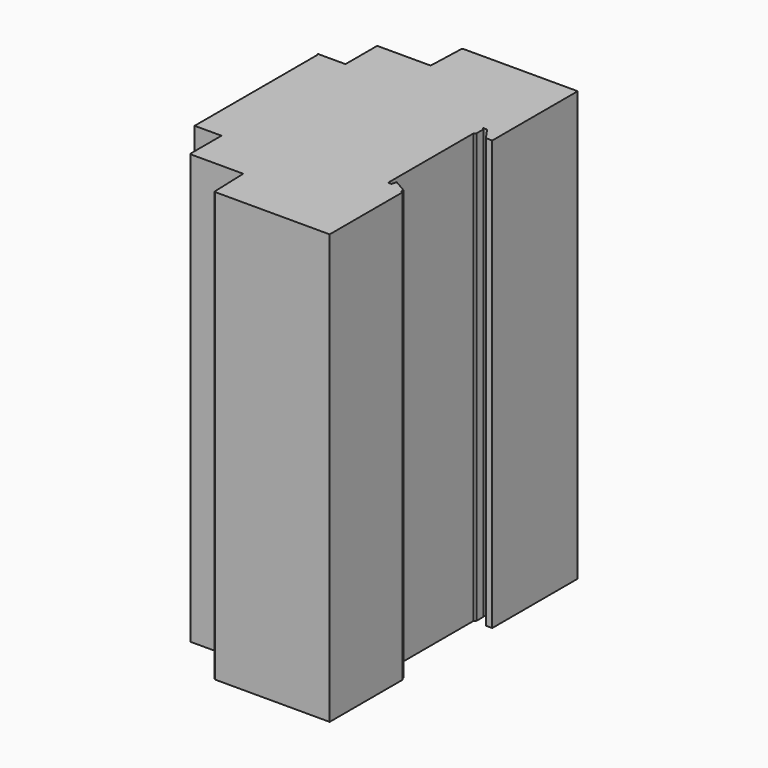
from build123d import *

# Parameters (mm, degrees)
F1_DEPTH = 124.6
F2_R     = 0.25
F3_R     = 2.1
F4_R     = 2.1
F6_DEPTH = 16
F5_W     = 44.5
F5_H     = 124.6
F5_W_2   = 30.3
F5_H_2   = 57.1
F5_R     = 3.57
F5_R_2   = 1
F5_W_3   = 24
F5_H_3   = 48
F5_R_3   = 2.35
F7_DEPTH = 0.2
F8_DEPTH = 0.5
F9_DEPTH = 0.1
F10_R    = 0.1


# Not quite as in the source:
# - ends of sketch curves that miss each other by under 0.0002 mm in the source are joined


with BuildPart() as f1:
    # F0 (on Top) → F1 (new body)
    with BuildSketch(Plane.XY):
        with BuildLine():
            ThreePointArc((-15.8128712425, -37.7039390085), (-15.7214514538, -37.9092709955), (-15.513054, -37.993469))
            Line((-15.513054, -37.993469), (4.69724, -37.993469))
            Line((4.69724, -37.993469), (5.19724, -37.993469))
            Line((5.19724, -37.993469), (17.69724, -37.993469))
            Line((17.69724, -37.993469), (17.69724, -11.597317))
            Line((17.69724, -11.597317), (17.19724, -11.463342))
            Line((17.19724, -11.463342), (17.19724, -10.586289))
            Line((17.19724, -10.586289), (13.572369, -8.493469))
            Line((13.572369, -8.493469), (13.19724, -9.893469))
            Line((13.19724, -9.893469), (12.19724, -9.893469))
            Line((12.19724, -9.893469), (12.19724, 21.006531))
            Line((12.19724, 21.006531), (12.69724, 21.506531))
            Line((12.69724, 21.506531), (12.69724, 24.006531))
            Line((12.69724, 24.006531), (12.19724, 24.506531))
            Line((12.19724, 24.506531), (13.39724, 24.506531))
            Line((13.39724, 24.506531), (15.847966, 21.006531))
            Line((15.847966, 21.006531), (17.69724, 21.006531))
            Line((17.69724, 21.006531), (17.69724, 52.006531))
            Line((17.69724, 52.006531), (-15.513054, 52.006531))
            ThreePointArc((-15.513054, 52.006531), (-15.7214514538, 51.9223329955), (-15.8128712425, 51.7170010085))
            Line((-15.8128712425, 51.7170010085), (-16.186889, 41.006531))
            Line((-16.186889, 41.006531), (-31.40276, 41.006531))
            ThreePointArc((-31.40276, 41.006531), (-31.6148920344, 40.9186630344), (-31.70276, 40.706531))
            Line((-31.70276, 40.706531), (-31.70276, 29.506531))
            Line((-31.70276, 29.506531), (-39.395956, 29.506531))
            Line((-39.395956, 29.506531), (-39.70276, 29.506531))
            Line((-39.70276, 29.506531), (-39.70276, 29.206531))
            Line((-39.70276, 29.206531), (-39.70276, -15.193469))
            Line((-39.70276, -15.193469), (-39.70276, -15.493469))
            Line((-39.70276, -15.493469), (-39.395956, -15.493469))
            Line((-39.395956, -15.493469), (-31.70276, -15.493469))
            Line((-31.70276, -15.493469), (-31.70276, -26.693469))
            ThreePointArc((-31.70276, -26.693469), (-31.6148920344, -26.9056010344), (-31.40276, -26.993469))
            Line((-31.40276, -26.993469), (-16.186889, -26.993469))
            Line((-16.186889, -26.993469), (-15.8128712425, -37.7039390085))
        make_face()
    extrude(amount=F1_DEPTH)

    # F2
    f2_edges = [f1.edges().sort_by_distance(p)[0] for p in [
        (-39.70276, -15.493469, 62.3),
        (-39.70276, 29.506531, 62.3),
    ]]
    fillet(f2_edges, radius=F2_R)

    # F3 (on face) + F4 (on face) → F6 (cut)
    with BuildSketch(Plane(origin=(-17.597409819, 0.6145153318, 0), x_dir=(-0.0348995103, -0.9993908265, 0), z_dir=(-0.9993908265, 0.0348995103, 0))):
        with Locations((-43.8236349213, 17.26)):
            Circle(F3_R)
        with Locations((-43.8236349213, 12.26)):
            Circle(F3_R)
        with Locations((-43.8236349213, 27.4)):
            Circle(F3_R)
        with Locations((-43.8236349213, 32.48)):
            Circle(F3_R)
        with Locations((-43.8236349213, 37.56)):
            Circle(F3_R)
        with Locations((-43.8236349213, 47.72)):
            Circle(F3_R)
        with Locations((-43.8236349213, 52.8)):
            Circle(F3_R)
        with Locations((-43.8236349213, 57.88)):
            Circle(F3_R)
        with Locations((-43.8236349213, 62.96)):
            Circle(F3_R)
        with Locations((-43.8236349213, 68.04)):
            Circle(F3_R)
        with Locations((-43.8236349213, 73.12)):
            Circle(F3_R)
        with Locations((-43.8236349213, 78.2)):
            Circle(F3_R)
        with Locations((-43.8236349213, 83.28)):
            Circle(F3_R)
        with Locations((-43.8236349213, 88.36)):
            Circle(F3_R)
        with Locations((-43.8236349213, 93.44)):
            Circle(F3_R)
    with BuildSketch(Plane(origin=(-17.108658733, -0.5974477611, 0), x_dir=(0.0348995103, -0.9993908265, 0), z_dir=(-0.9993908265, -0.0348995103, 0))):
        with Locations((29.8289263992, 5.64)):
            Circle(F4_R)
        with Locations((29.8289263992, 10.68)):
            Circle(F4_R)
        with Locations((29.8289263992, 20.84)):
            Circle(F4_R)
        with Locations((29.8289263992, 25.92)):
            Circle(F4_R)
        with Locations((29.8289263992, 33)):
            Circle(F4_R)
        with Locations((29.8289263992, 38.08)):
            Circle(F4_R)
        with Locations((29.8289263992, 48.24)):
            Circle(F4_R)
        with Locations((29.8289263992, 53.32)):
            Circle(F4_R)
        with Locations((29.8289263992, 60.4)):
            Circle(F4_R)
        with Locations((29.8289263992, 65.48)):
            Circle(F4_R)
        with Locations((29.8289263992, 75.64)):
            Circle(F4_R)
        with Locations((29.8289263992, 80.72)):
            Circle(F4_R)
        with Locations((29.8289263992, 87.8)):
            Circle(F4_R)
        with Locations((29.8289263992, 92.88)):
            Circle(F4_R)
        with Locations((29.8289263992, 103.04)):
            Circle(F4_R)
        with Locations((29.8289263992, 108.12)):
            Circle(F4_R)
    extrude(amount=-F6_DEPTH, dir=(-0.9993908265, 0.0348995103, 0), mode=Mode.SUBTRACT)

    # F5 (on face) → F7 (cut)
    with BuildSketch(Plane(origin=(-39.70276, 0, 0), x_dir=(0, -1, 0), z_dir=(-1, 0, 0))):
        with Locations((-7.006531, 62.3)):
            Rectangle(F5_W, F5_H)
        with Locations((-10.906531, 28.85)):
            Rectangle(F5_W_2, F5_H_2, mode=Mode.SUBTRACT)
        with Locations((9.493469, 9.42)):
            Circle(F5_R, mode=Mode.SUBTRACT)
        with Locations((9.493469, 19.62)):
            Circle(F5_R, mode=Mode.SUBTRACT)
        with Locations((9.493469, 29.82)):
            Circle(F5_R, mode=Mode.SUBTRACT)
        with Locations((9.493469, 40.02)):
            Circle(F5_R, mode=Mode.SUBTRACT)
        with Locations((9.493469, 50.22)):
            Circle(F5_R, mode=Mode.SUBTRACT)
        with Locations((-21.946531, 83.29)):
            Circle(F5_R_2, mode=Mode.SUBTRACT)
        with Locations((-21.946531, 93.29)):
            Circle(F5_R_2, mode=Mode.SUBTRACT)
        with Locations((-11.946531, 83.29)):
            Circle(F5_R_2, mode=Mode.SUBTRACT)
        with Locations((-11.946531, 93.29)):
            Circle(F5_R_2, mode=Mode.SUBTRACT)
        with Locations((-21.946531, 103.29)):
            Circle(F5_R_2, mode=Mode.SUBTRACT)
        with Locations((-21.946531, 113.29)):
            Circle(F5_R_2, mode=Mode.SUBTRACT)
        with Locations((-11.946531, 103.29)):
            Circle(F5_R_2, mode=Mode.SUBTRACT)
        with Locations((-11.946531, 113.29)):
            Circle(F5_R_2, mode=Mode.SUBTRACT)
        with Locations((-1.946531, 83.29)):
            Circle(F5_R_2, mode=Mode.SUBTRACT)
        with Locations((-1.946531, 93.29)):
            Circle(F5_R_2, mode=Mode.SUBTRACT)
        with Locations((9.493469, 64.82)):
            Circle(F5_R, mode=Mode.SUBTRACT)
        with Locations((8.053469, 83.29)):
            Circle(F5_R_2, mode=Mode.SUBTRACT)
        with Locations((8.053469, 93.29)):
            Circle(F5_R_2, mode=Mode.SUBTRACT)
        with Locations((-1.946531, 103.29)):
            Circle(F5_R_2, mode=Mode.SUBTRACT)
        with Locations((-1.946531, 113.29)):
            Circle(F5_R_2, mode=Mode.SUBTRACT)
        with Locations((8.053469, 103.29)):
            Circle(F5_R_2, mode=Mode.SUBTRACT)
        with Locations((8.053469, 113.29)):
            Circle(F5_R_2, mode=Mode.SUBTRACT)
        with Locations((-10.906531, 28.85)):
            Rectangle(F5_W_2, F5_H_2)
        with Locations((-10.906531, 29.8)):
            Rectangle(F5_W_3, F5_H_3, mode=Mode.SUBTRACT)
        with Locations((-10.906531, 29.8)):
            Rectangle(F5_W_3, F5_H_3)
        with Locations((9.493469, 9.42)):
            Circle(F5_R)
        with Locations((9.493469, 9.42)):
            Circle(F5_R_3, mode=Mode.SUBTRACT)
        with Locations((9.493469, 19.62)):
            Circle(F5_R)
        with Locations((9.493469, 19.62)):
            Circle(F5_R_3, mode=Mode.SUBTRACT)
        with Locations((9.493469, 29.82)):
            Circle(F5_R)
        with Locations((9.493469, 29.82)):
            Circle(F5_R_3, mode=Mode.SUBTRACT)
        with Locations((9.493469, 40.02)):
            Circle(F5_R)
        with Locations((9.493469, 40.02)):
            Circle(F5_R_3, mode=Mode.SUBTRACT)
        with Locations((9.493469, 50.22)):
            Circle(F5_R)
        with Locations((9.493469, 50.22)):
            Circle(F5_R_3, mode=Mode.SUBTRACT)
        with Locations((9.493469, 64.82)):
            Circle(F5_R)
        with Locations((9.493469, 64.82)):
            Circle(F5_R_3, mode=Mode.SUBTRACT)
        with Locations((-21.946531, 83.29)):
            Circle(F5_R_2)
        with Locations((-21.946531, 93.29)):
            Circle(F5_R_2)
        with Locations((-21.946531, 103.29)):
            Circle(F5_R_2)
        with Locations((-21.946531, 113.29)):
            Circle(F5_R_2)
        with Locations((-11.946531, 113.29)):
            Circle(F5_R_2)
        with Locations((-11.946531, 103.29)):
            Circle(F5_R_2)
        with Locations((-11.946531, 93.29)):
            Circle(F5_R_2)
        with Locations((-11.946531, 83.29)):
            Circle(F5_R_2)
        with Locations((-1.946531, 83.29)):
            Circle(F5_R_2)
        with Locations((-1.946531, 93.29)):
            Circle(F5_R_2)
        with Locations((-1.946531, 103.29)):
            Circle(F5_R_2)
        with Locations((-1.946531, 113.29)):
            Circle(F5_R_2)
        with Locations((8.053469, 113.29)):
            Circle(F5_R_2)
        with Locations((8.053469, 103.29)):
            Circle(F5_R_2)
        with Locations((8.053469, 93.29)):
            Circle(F5_R_2)
        with Locations((8.053469, 83.29)):
            Circle(F5_R_2)
    extrude(amount=-F7_DEPTH, mode=Mode.SUBTRACT)

    # F5 (on face) → F8 (cut)
    with BuildSketch(Plane(origin=(-39.70276, 0, 0), x_dir=(0, -1, 0), z_dir=(-1, 0, 0))):
        with Locations((-10.906531, 29.8)):
            Rectangle(F5_W_3, F5_H_3)
        with Locations((-21.946531, 83.29)):
            Circle(F5_R_2)
        with Locations((-21.946531, 93.29)):
            Circle(F5_R_2)
        with Locations((-21.946531, 103.29)):
            Circle(F5_R_2)
        with Locations((-11.946531, 83.29)):
            Circle(F5_R_2)
        with Locations((-11.946531, 93.29)):
            Circle(F5_R_2)
        with Locations((-11.946531, 103.29)):
            Circle(F5_R_2)
        with Locations((-1.946531, 83.29)):
            Circle(F5_R_2)
        with Locations((-1.946531, 93.29)):
            Circle(F5_R_2)
        with Locations((8.053469, 83.29)):
            Circle(F5_R_2)
        with Locations((8.053469, 93.29)):
            Circle(F5_R_2)
        with Locations((-1.946531, 103.29)):
            Circle(F5_R_2)
        with Locations((8.053469, 103.29)):
            Circle(F5_R_2)
        with Locations((8.053469, 113.29)):
            Circle(F5_R_2)
        with Locations((-1.946531, 113.29)):
            Circle(F5_R_2)
        with Locations((-11.946531, 113.29)):
            Circle(F5_R_2)
        with Locations((-21.946531, 113.29)):
            Circle(F5_R_2)
    extrude(amount=-F8_DEPTH, mode=Mode.SUBTRACT)

    # F10
    f10_edges = [f1.edges().sort_by_distance(p)[0] for p in [
        (-39.70276, -15.243469, 62.3),
        (-39.70276, 29.256531, 62.3),
    ]]
    fillet(f10_edges, radius=F10_R)


with BuildPart() as f9:
    # F5 (on face) → F9 (new body)
    with BuildSketch(Plane(origin=(-39.70276, 0, 0), x_dir=(0, -1, 0), z_dir=(-1, 0, 0))):
        with Locations((-10.906531, 28.85)):
            Rectangle(F5_W_2, F5_H_2)
        with Locations((-10.906531, 29.8)):
            Rectangle(F5_W_3, F5_H_3, mode=Mode.SUBTRACT)
    extrude(amount=F9_DEPTH)


solid = Compound([f1.part, f9.part])
